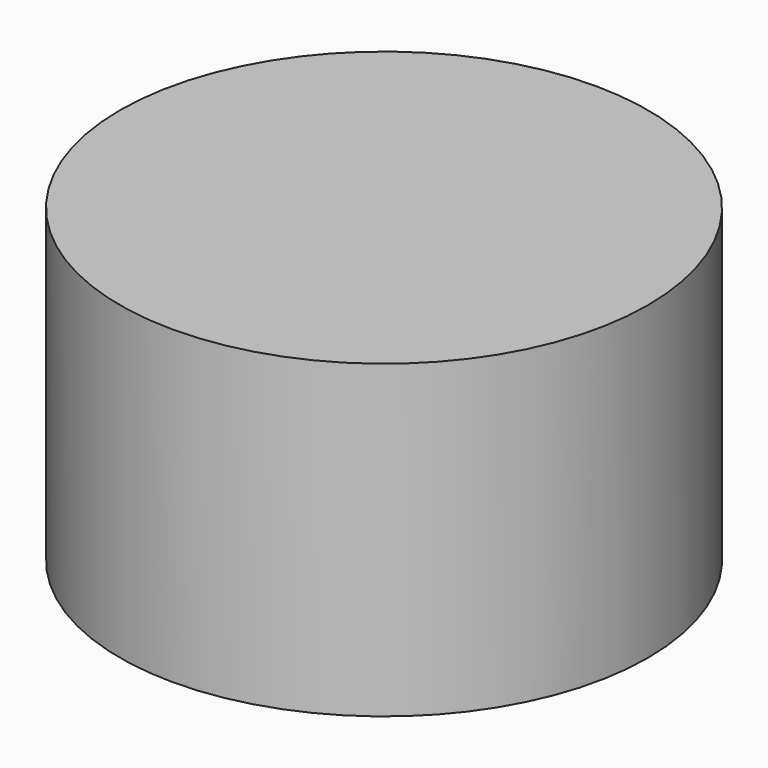
from build123d import *

# Parameters (mm, degrees)
F0_R     = 21.2543293748
F1_DEPTH = 25


# Not quite as in the source:
# - the program builds the solid bodies; features that only make, move or delete a surface that nothing else refers to are left out


with BuildPart() as f1:
    # F0 (on Top) → F1 (new body)
    with BuildSketch(Plane.XY):
        Circle(F0_R)
    extrude(amount=F1_DEPTH)


solid = f1.part
